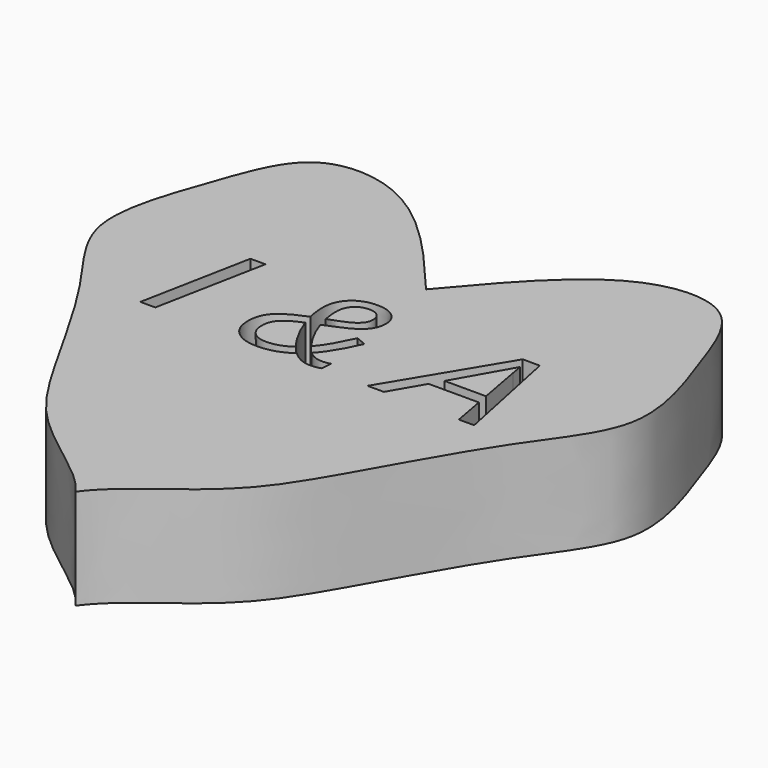
from build123d import *

# Parameters (mm, degrees)
F1_DEPTH     = 10
F2_TEXT_SIZE = 16.0320641283
F3_DEPTH     = 5


# Not quite as in the source:
# - Text() gives the source's letters only with a copy of the font that has no kerning and outlines rounded to 1/6400 em; it was checked with that copy


with BuildPart() as f1:
    # F0 (on Top) → F1 (new body)
    with BuildSketch(Plane.XY):
        with BuildLine():
            add(Edge.make_bspline(
                [(0, 13.4655078873), (3.8495567471, 18.0372501237), (10.425747561, 25.8471491002), (21.2295174882, 26.2841995295), (24.3244527866, 17.0464876408), (28.4225252268, 5.8548936388), (21.0684515734, -2.3897823144), (13.7248062956, -16.4494050892), (9.299597009, -22.7320460539), (1.785158616, -27.8562496306), (0.474346148, -29.5635024517), (0, -30.1813092083)],
                knots=[0, 0, 0, 0, 0.1451224383, 0.2479123982, 0.354147106, 0.4733901908, 0.5892824489, 0.7318987489, 0.8349135122, 0.9402598454, 1, 1, 1, 1], degree=3))
            add(Edge.make_bspline(
                [(0, 13.4655078873), (-3.8495567471, 18.0372501237), (-10.425747561, 25.8471491002), (-21.2295174882, 26.2841995295), (-24.3244527866, 17.0464876408), (-28.4225252268, 5.8548936388), (-21.0684515734, -2.3897823144), (-13.7248062956, -16.4494050892), (-9.299597009, -22.7320460539), (-1.785158616, -27.8562496306), (-0.474346148, -29.5635024517), (0, -30.1813092083)],
                knots=[0, 0, 0, 0, 0.1451224383, 0.2479123982, 0.354147106, 0.4733901908, 0.5892824489, 0.7318987489, 0.8349135122, 0.9402598454, 1, 1, 1, 1], degree=3))
        make_face()
    extrude(amount=F1_DEPTH)

    # F2 (on face) → F3 (cut)
    with BuildSketch(Plane.XY.offset(10)):
        with Locations((-16.6667756281, -2.0716679642)):
            Text('I & A', F2_TEXT_SIZE, font='Arimo', font_style=FontStyle.ITALIC, text_align=(TextAlign.LEFT, TextAlign.BOTTOM))
    extrude(amount=-F3_DEPTH, mode=Mode.SUBTRACT)


solid = f1.part
